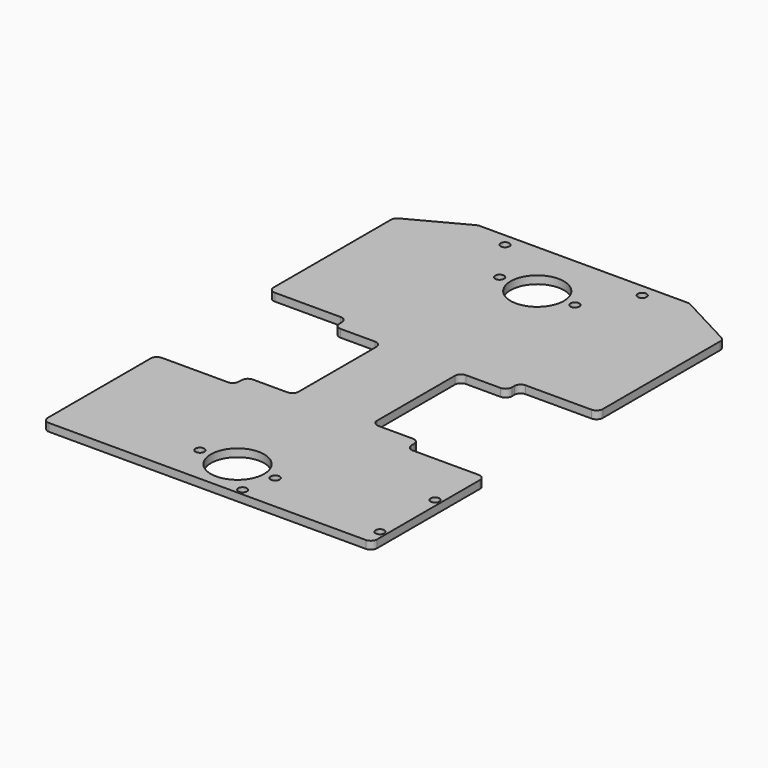
from build123d import *

# Parameters (mm, degrees)
F0_R     = 1.7859375
F0_R_2   = 10.795
F1_DEPTH = 3.175
F2_R     = 2.54


with BuildPart() as f1:
    # F0 (on Top) → F1 (new body)
    with BuildSketch(Plane.XY):
        Polygon((-136.4652514458, -19.908263123), (-136.4652514458, -77.058263123), (-3.1152514458, -77.058263123), (-3.1152514458, -19.908263123), (-34.8652514458, -19.908263123), (-34.8652514458, -13.558263123), (-53.9152514458, -13.558263123), (-53.9152514458, 30.891736877), (-34.8652514458, 30.891736877), (-34.8652514458, 37.241736877), (-3.1152514458, 37.241736877), (-3.1152514458, 100.741736877), (-27.0015158653, 113.441736877), (-112.5789870262, 113.441736877), (-136.4652514458, 100.741736877), (-136.4652514458, 37.241736877), (-104.7152514458, 37.241736877), (-104.7152514458, 30.891736877), (-85.6652514458, 30.891736877), (-85.6652514458, -13.558263123), (-104.7152514458, -13.558263123), (-104.7152514458, -19.908263123), align=None)
        with Locations((-85.0302514458, -61.818263123)):
            Circle(F0_R, mode=Mode.SUBTRACT)
        with Locations((-57.5474514458, -74.569063123)):
            Circle(F0_R, mode=Mode.SUBTRACT)
        with Locations((-69.7902514458, -61.818263123)):
            Circle(F0_R_2, mode=Mode.SUBTRACT)
        with Locations((-54.5502514458, -61.818263123)):
            Circle(F0_R, mode=Mode.SUBTRACT)
        with Locations((-5.6552514458, -69.870063123)):
            Circle(F0_R, mode=Mode.SUBTRACT)
        with Locations((-5.6552514458, -41.980863123)):
            Circle(F0_R, mode=Mode.SUBTRACT)
        with Locations((-97.5715014458, 108.361736877)):
            Circle(F0_R, mode=Mode.SUBTRACT)
        with Locations((-85.0302514458, 89.946736877)):
            Circle(F0_R, mode=Mode.SUBTRACT)
        with Locations((-69.7902514458, 89.946736877)):
            Circle(F0_R_2, mode=Mode.SUBTRACT)
        with Locations((-54.5502514458, 89.946736877)):
            Circle(F0_R, mode=Mode.SUBTRACT)
        with Locations((-42.0090014458, 108.361736877)):
            Circle(F0_R, mode=Mode.SUBTRACT)
    extrude(amount=F1_DEPTH)

    # F2
    f2_edges = [f1.edges().sort_by_distance(p)[0] for p in [
        (-34.865251, 37.241737, 1.5875),
        (-3.115251, -19.908263, 1.5875),
        (-3.115251, 37.241737, 1.5875),
        (-3.115251, -77.058263, 1.5875),
        (-136.465251, -77.058263, 1.5875),
        (-3.115251, 100.741737, 1.5875),
        (-27.001516, 113.441737, 1.5875),
        (-112.578987, 113.441737, 1.5875),
        (-136.465251, 100.741737, 1.5875),
        (-136.465251, 37.241737, 1.5875),
        (-104.715251, 37.241737, 1.5875),
        (-136.465251, -19.908263, 1.5875),
        (-53.915251, 30.891737, 1.5875),
        (-53.915251, -13.558263, 1.5875),
        (-85.665251, -13.558263, 1.5875),
        (-104.715251, -13.558263, 1.5875),
        (-85.665251, 30.891737, 1.5875),
        (-34.865251, -13.558263, 1.5875),
        (-104.715251, 30.891737, 1.5875),
        (-104.715251, -19.908263, 1.5875),
        (-34.865251, -19.908263, 1.5875),
        (-34.865251, 30.891737, 1.5875),
    ]]
    fillet(f2_edges, radius=F2_R)


solid = f1.part
